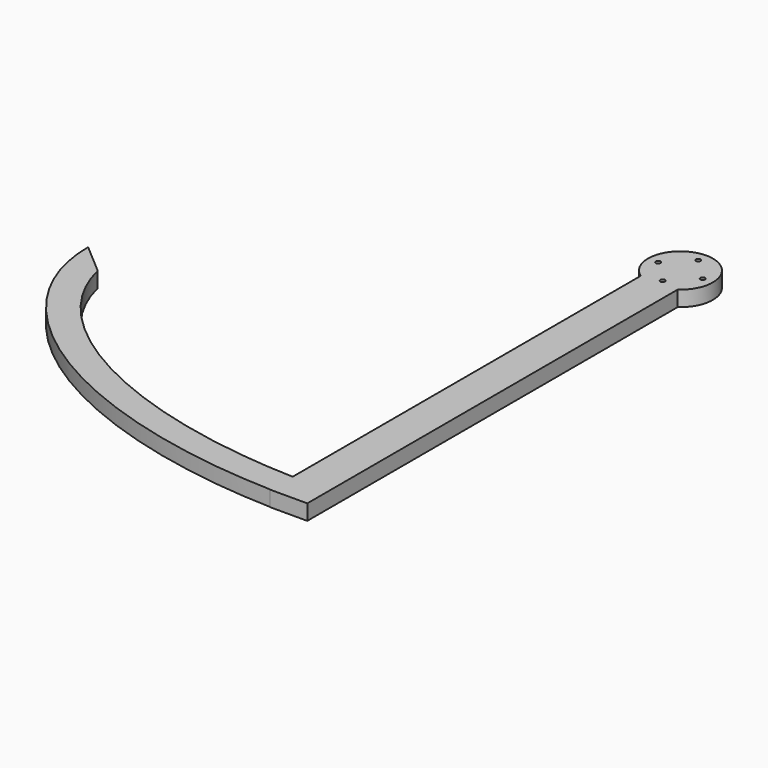
from build123d import *

# Parameters (mm, degrees)
F0_R     = 10.5
F0_R_2   = 0.75
F1_DEPTH = 5
F3_DEPTH = 5


# Not quite as in the source:
# - a feature names something its author has since deleted; it is built from what else it names


with BuildPart() as f1:
    # F0 (on Top) → F1 (new body)
    with BuildSketch(Plane.XY):
        Circle(F0_R)
        with Locations((-3.45, -7.2)):
            Circle(F0_R_2, mode=Mode.SUBTRACT)
        with Locations((-7.2, -3.45)):
            Circle(F0_R_2, mode=Mode.SUBTRACT)
        with Locations((0, -7.2)):
            Circle(F0_R_2, mode=Mode.SUBTRACT)
        with Locations((3.45, -7.2)):
            Circle(F0_R_2, mode=Mode.SUBTRACT)
        with Locations((7.2, -3.45)):
            Circle(F0_R_2, mode=Mode.SUBTRACT)
        with Locations((-7.2, 0)):
            Circle(F0_R_2, mode=Mode.SUBTRACT)
        with Locations((-7.2, 3.45)):
            Circle(F0_R_2, mode=Mode.SUBTRACT)
        with Locations((-3.45, 7.2)):
            Circle(F0_R_2, mode=Mode.SUBTRACT)
        with Locations((7.2, 0)):
            Circle(F0_R_2, mode=Mode.SUBTRACT)
        with Locations((7.2, 3.45)):
            Circle(F0_R_2, mode=Mode.SUBTRACT)
        with Locations((0, 7.2)):
            Circle(F0_R_2, mode=Mode.SUBTRACT)
        with Locations((3.45, 7.2)):
            Circle(F0_R_2, mode=Mode.SUBTRACT)
        with Locations((3.45, -7.2)):
            Circle(F0_R_2)
        with Locations((-3.45, -7.2)):
            Circle(F0_R_2)
        with Locations((-7.2, -3.45)):
            Circle(F0_R_2)
        with Locations((-7.2, 3.45)):
            Circle(F0_R_2)
        with Locations((-3.45, 7.2)):
            Circle(F0_R_2)
        with Locations((3.45, 7.2)):
            Circle(F0_R_2)
        with Locations((7.2, 3.45)):
            Circle(F0_R_2)
        with Locations((7.2, -3.45)):
            Circle(F0_R_2)
    extrude(amount=F1_DEPTH)

    # F2 (on Top) → F3 (join, through all)
    with BuildSketch(Plane.XY):
        with BuildLine():
            Line((6, -8.7032937936), (6, -8.6168439698))
            Line((6, -8.6168439698), (-5.159e-07, -8.6168439698))
            add(Edge.make_bspline(
                [(6, -8.7032937936), (3.0017297357, -8.6168439624), (-5.159e-07, -8.6168439698)],
                knots=[4.6643705292, 4.6643705292, 4.6643705292, 4.7123889845, 4.7123889845, 4.7123889845], degree=2, weights=[1, 0.9997117923, 1]))
        make_face()
        with BuildLine():
            add(Edge.make_bspline(
                [(-5.159e-07, -8.6168439698), (-3.0017302513, -8.6168439772), (-6, -8.7032937936)],
                knots=[4.7123889845, 4.7123889845, 4.7123889845, 4.7604074315, 4.7604074315, 4.7604074315], degree=2, weights=[1, 0.9997117924, 1]))
            Line((-5.159e-07, -8.6168439698), (-6, -8.6168439698))
            Line((-6, -8.6168439698), (-6, -8.7032937936))
        make_face()
        with BuildLine():
            Line((6, -158.6168439698), (6, -158.530394146))
            add(Edge.make_bspline(
                [(0, -158.6168439698), (3.0017299935, -158.6168439698), (6, -158.530394146)],
                knots=[1.5707963268, 1.5707963268, 1.5707963268, 1.6188147779, 1.6188147779, 1.6188147779], degree=2, weights=[1, 0.9997117924, 1]))
            Line((0, -158.6168439698), (6, -158.6168439698))
        make_face()
        with BuildLine():
            Line((-6, -158.6168439698), (0, -158.6168439698))
            add(Edge.make_bspline(
                [(-6, -158.530394146), (-3.0017299935, -158.6168439698), (0, -158.6168439698)],
                knots=[1.5227778757, 1.5227778757, 1.5227778757, 1.5707963268, 1.5707963268, 1.5707963268], degree=2, weights=[1, 0.9997117924, 1]))
            Line((-6, -158.530394146), (-6, -158.6168439698))
        make_face()
        with BuildLine():
            add(Edge.make_bspline(
                [(0, -158.6168439698), (3.0017299935, -158.6168439698), (6, -158.530394146)],
                knots=[1.5707963268, 1.5707963268, 1.5707963268, 1.6188147779, 1.6188147779, 1.6188147779], degree=2, weights=[1, 0.9997117924, 1]))
            Line((6, -158.530394146), (6, -149.528497087))
            add(Edge.make_bspline(
                [(-6, -149.528497087), (0, -149.7053092713), (6, -149.528497087)],
                knots=[1.5190490974, 1.5190490974, 1.5190490974, 1.6225435562, 1.6225435562, 1.6225435562], degree=2, weights=[1, 0.9986614109, 1]))
            Line((-6, -149.528497087), (-6, -158.530394146))
            add(Edge.make_bspline(
                [(-6, -158.530394146), (-3.0017299935, -158.6168439698), (0, -158.6168439698)],
                knots=[1.5227778757, 1.5227778757, 1.5227778757, 1.5707963268, 1.5707963268, 1.5707963268], degree=2, weights=[1, 0.9997117924, 1]))
        make_face()
        with BuildLine():
            add(Edge.make_bspline(
                [(6, -8.7032937936), (3.0017297357, -8.6168439624), (-5.159e-07, -8.6168439698)],
                knots=[4.6643705292, 4.6643705292, 4.6643705292, 4.7123889845, 4.7123889845, 4.7123889845], degree=2, weights=[1, 0.9997117923, 1]))
            add(Edge.make_bspline(
                [(-5.159e-07, -8.6168439698), (-3.0017302513, -8.6168439772), (-6, -8.7032937936)],
                knots=[4.7123889845, 4.7123889845, 4.7123889845, 4.7604074315, 4.7604074315, 4.7604074315], degree=2, weights=[1, 0.9997117924, 1]))
            Line((-6, -8.7032937936), (-6, -17.7051908526))
            add(Edge.make_bspline(
                [(6, -17.7051908526), (0, -17.5283786684), (-6, -17.7051908526)],
                knots=[4.660641751, 4.660641751, 4.660641751, 4.7641362098, 4.7641362098, 4.7641362098], degree=2, weights=[1, 0.9986614109, 1]))
            Line((6, -17.7051908526), (6, -8.7032937936))
        make_face()
        with BuildLine():
            Line((6, -149.528497087), (6, -17.7051908526))
            add(Edge.make_bspline(
                [(6, -17.7051908526), (0, -17.5283786684), (-6, -17.7051908526)],
                knots=[4.660641751, 4.660641751, 4.660641751, 4.7641362098, 4.7641362098, 4.7641362098], degree=2, weights=[1, 0.9986614109, 1]))
            Line((-6, -17.7051908526), (-6, -149.528497087))
            add(Edge.make_bspline(
                [(-6, -149.528497087), (0, -149.7053092713), (6, -149.528497087)],
                knots=[1.5190490974, 1.5190490974, 1.5190490974, 1.6225435562, 1.6225435562, 1.6225435562], degree=2, weights=[1, 0.9986614109, 1]))
        make_face()
        with BuildLine():
            Line((-115.0107222667, -92.2180852847), (-125, -83.6168439698))
            add(Edge.make_bspline(
                [(-125, -83.6168439698), (-125, -155.0992391761), (-6, -158.530394146)],
                knots=[0, 0, 0, 1.5227778757, 1.5227778757, 1.5227778757], degree=2, weights=[1, 0.7238784428, 1]))
            Line((-6, -158.530394146), (-6, -149.528497087))
            add(Edge.make_bspline(
                [(-115.0107222667, -92.2180852847), (-102.427295797, -146.686910289), (-6, -149.528497087)],
                knots=[0.1306935792, 0.1306935792, 0.1306935792, 1.5190490974, 1.5190490974, 1.5190490974], degree=2, weights=[1, 0.7685799932, 1]))
        make_face()
    extrude(amount=F3_DEPTH)


solid = f1.part
